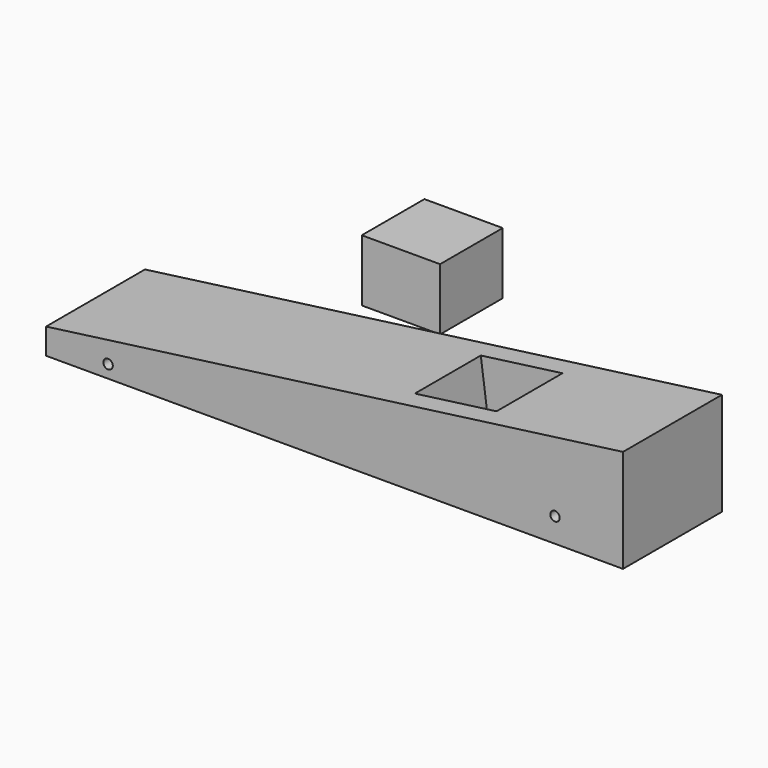
from build123d import *

# Parameters (mm, degrees)
F1_DEPTH  = 38.1
F2_W      = 25.4
F2_H      = 25.4
F4_DEPTH  = 19.05
F6_R      = 1.4605
F7_DEPTH  = 38.1
F9_R      = 1.4605
F10_DEPTH = 38.1
F12_W     = 24.13
F12_H     = 24.13
F13_DEPTH = 19.05


# Not quite as in the source:
# - a feature of the source that left no trace in its solid (it failed there, or was rolled back) is left out


with BuildPart() as f1:
    # F0 (on Front) → F1 (new body)
    with BuildSketch(Plane.XZ):
        Polygon((96.6367053866, 0.1098374724), (96.6367053866, 31.8598374724), (-81.1632946134, 8.0473374724), (-81.1632946134, 0.1098374724), align=None)
    extrude(amount=F1_DEPTH)

    # F2 (on face) → F4 (cut)
    with BuildSketch(Plane(origin=(-2.4889394817, 0, 18.5840814633), x_dir=(0.9911504425, 0, 0.1327433628), z_dir=(-0.1327433628, 0, 0.9911504425))):
        with Locations((42.8606952689, -19.05)):
            Rectangle(F2_W, F2_H)
    extrude(amount=-F4_DEPTH, mode=Mode.SUBTRACT)

    # F6 (on face) → F7 (cut)
    with BuildSketch(Plane.XZ.offset(38.1)):
        with Locations((-62.0626753688, 4.064)):
            Circle(F6_R)
    extrude(amount=-F7_DEPTH, mode=Mode.SUBTRACT)

    # F9 (on face) → F10 (cut)
    with BuildSketch(Plane.XZ.offset(38.1)):
        with Locations((75.6781622767, 7.5987153687)):
            Circle(F9_R)
    extrude(amount=-F10_DEPTH, mode=Mode.SUBTRACT)


with BuildPart() as f13:
    # F12 (on Top) → F13 (new body)
    with BuildSketch(Plane.XY):
        with Locations((-26.2855645269, 42.0638084072)):
            Rectangle(F12_W, F12_H)
    extrude(amount=F13_DEPTH)


solid = Compound([f1.part, f13.part])
